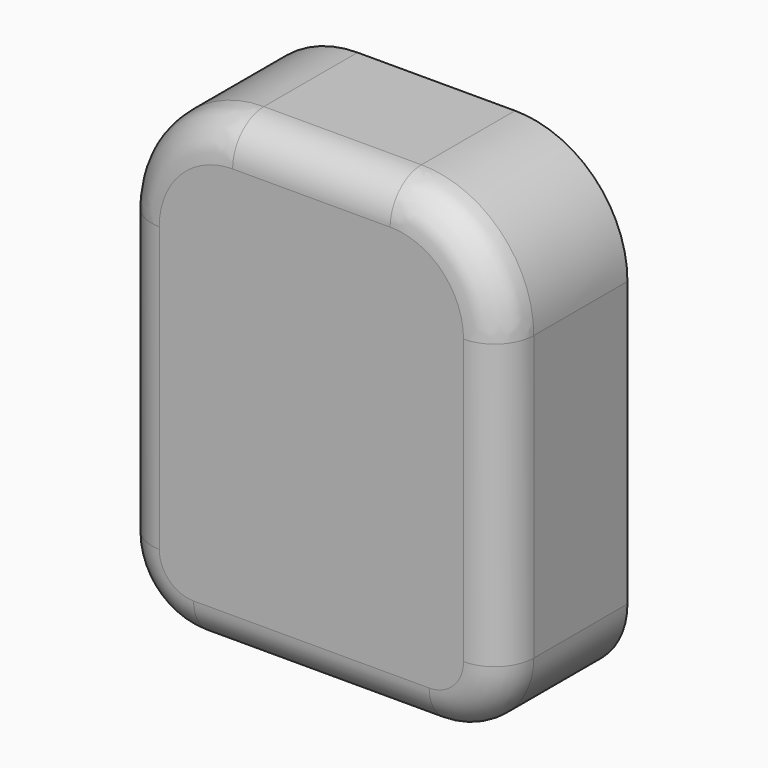
from build123d import *

# Parameters (mm, degrees)
F1_DEPTH = 2
F2_R     = 0.5


with BuildPart() as f1:
    # F0 (on Front) → F1 (new body)
    with BuildSketch(Plane.XZ):
        with BuildLine():
            Line((2.5171569428, -2.0559416641), (2.5171569428, 1.5825099279))
            add(Edge.make_bspline(
                [(2.5171569428, 1.5825099279), (2.5171569428, 1.6787899754), (2.4992681155, 1.8667750179), (2.4168759633, 2.1410945762), (2.2843862606, 2.3947087975), (2.105016137, 2.616022741), (1.8857868809, 2.8002460755), (1.636045778, 2.935551434), (1.3611822969, 3.0213954134), (1.1734702016, 3.0397964861), (1.077156934, 3.0397964861)],
                knots=[0, 0, 0, 0, 0.125, 0.25, 0.375, 0.5, 0.625, 0.75, 0.875, 1, 1, 1, 1], degree=3))
            Line((1.077156934, 3.0397964861), (-0.9413276869, 3.0397964861))
            add(Edge.make_bspline(
                [(-0.9413276869, 3.0397964861), (-1.0374200662, 3.0397964861), (-1.2247764123, 3.021445425), (-1.4988313624, 2.9361167775), (-1.7490503253, 2.8008991891), (-1.9684911225, 2.6167308737), (-2.1479113142, 2.3956347723), (-2.2804861743, 2.1425165112), (-2.363389349, 1.8673649273), (-2.3813276957, 1.6790159091), (-2.3813276957, 1.5825099279)],
                knots=[0, 0, 0, 0, 0.125, 0.25, 0.375, 0.5, 0.625, 0.75, 0.875, 1, 1, 1, 1], degree=3))
            Line((-2.3813276957, 1.5825099279), (-2.3813276957, -2.0559416641))
            ThreePointArc((-2.3813276957, -2.0559416641), (-2.1060080675, -2.7206220446), (-1.4413276869, -2.9959416729))
            Line((-1.4413276869, -2.9959416729), (1.577156934, -2.9959416729))
            ThreePointArc((1.577156934, -2.9959416729), (2.2418373145, -2.7206220446), (2.5171569428, -2.0559416641))
        make_face()
    extrude(amount=F1_DEPTH)

    # F2
    f2_edges = [f1.edges().sort_by_distance(p)[0] for p in [
        (-2.381328, -2, -0.236716),
        (0.067915, -2, -2.995942),
        (2.241837, -2, -2.720622),
        (2.517157, -2, -0.236716),
        (2.098373, -2, 2.609841),
        (0.067915, -2, 3.039796),
        (-1.961821, -2, 2.610576),
        (-2.106008, -2, -2.720622),
    ]]
    fillet(f2_edges, radius=F2_R)


solid = f1.part
